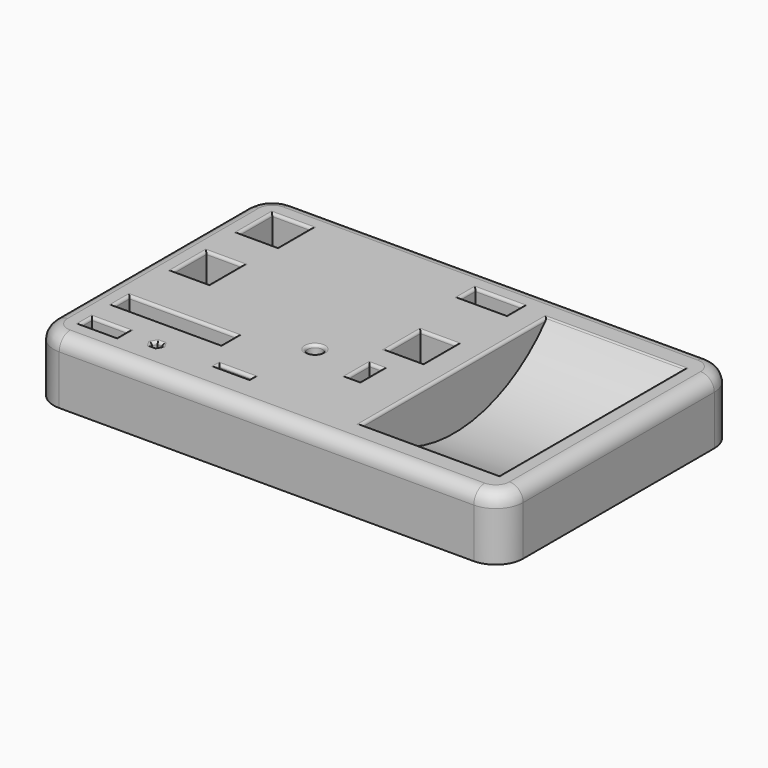
from build123d import *

# Parameters (mm, degrees)
F0_W          = 111
F0_H          = 107
F0_W_2        = 13
F0_H_2        = 5
F0_W_3        = 39
F0_H_3        = 7
F0_W_4        = 12
F0_H_4        = 1.5
F0_R          = 2.75
F0_W_5        = 4.5
F0_H_5        = 10
F0_H_6        = 15
F0_W_6        = 14
F0_W_7        = 17
F1_DEPTH      = 23
F2_W          = 111
F2_H          = 107
F3_DEPTH      = 3
F4_DEPTH      = 5
F5_DEPTH      = 13
F7_DEPTH      = 50
F9_DEPTH      = 10
F10_R         = 5
F11_T3_ANGLE  = 90
F11_T6_ANGLE  = 90
F11_T9_ANGLE  = 90
F11_T12_ANGLE = 90
F11_T15_DEPTH = 48
F11_T18_DEPTH = 48
F11_T21_DEPTH = 48
F11_T24_DEPTH = 48
F12_R         = 1


# Not quite as in the source:
# - a fillet or chamfer that OpenCascade refuses, or shapes differently, is made with other operations: its cross-section is extruded or revolved along the edge and cut away or added


with BuildPart() as f1:
    # F0 (on Top) → F1 (new body)
    with BuildSketch(Plane.XY):
        with Locations((55.5, 53.5)):
            Rectangle(F0_W, F0_H)
        with Locations((16.5, 12.5)):
            Rectangle(F0_W_2, F0_H_2, mode=Mode.SUBTRACT)
        Polygon((35.5980762114, 15), (36.4641016151, 13.5), (35.5980762114, 12), (33.8660254038, 12), (33, 13.5), (33.8660254038, 15), align=None, mode=Mode.SUBTRACT)
        with Locations((29.5, 28.5)):
            Rectangle(F0_W_3, F0_H_3, mode=Mode.SUBTRACT)
        with Locations((62.4641016151, 14.25)):
            Rectangle(F0_W_4, F0_H_4, mode=Mode.SUBTRACT)
        with Locations((71.75, 39.25)):
            Circle(F0_R, mode=Mode.SUBTRACT)
        with Locations((91.75, 37)):
            Rectangle(F0_W_5, F0_H_5, mode=Mode.SUBTRACT)
        with Locations((16.5, 59.5)):
            Rectangle(F0_W_2, F0_H_6, mode=Mode.SUBTRACT)
        with Locations((17, 89.5)):
            Rectangle(F0_W_6, F0_H_6, mode=Mode.SUBTRACT)
        with Locations((94.5, 59.5)):
            Rectangle(F0_W_2, F0_H_6, mode=Mode.SUBTRACT)
        with Locations((92.5, 93.5)):
            Rectangle(F0_W_7, F0_H_3, mode=Mode.SUBTRACT)
    extrude(amount=F1_DEPTH)

    # F2 (on face) → F3 (join)
    with BuildSketch(Plane(origin=(0, 0, 0), x_dir=(1, 0, 0), z_dir=(0, 0, -1))):
        with Locations((55.5, -53.5)):
            Rectangle(F2_W, F2_H)
    extrude(amount=-F3_DEPTH)

    # F4 (add): a face of the model
    f4_faces = [f1.faces().sort_by_distance(p)[0] for p in [
        (16.5, 12.5, 3),
    ]]
    extrude(f4_faces, amount=F4_DEPTH)

    # F5 (add): a face of the model
    f5_faces = [f1.faces().sort_by_distance(p)[0] for p in [
        (62.4641016151, 14.25, 3),
    ]]
    extrude(f5_faces, amount=F5_DEPTH)

    # F6 (on face) → F7 (join)
    with BuildSketch(Plane.YZ.offset(111)):
        with BuildLine():
            Line((11.0735931288, 23), (0, 23))
            Line((0, 23), (0, 0))
            Line((0, 0), (107, 0))
            Line((107, 0), (107, 23))
            Line((107, 23), (95.9264068712, 23))
            ThreePointArc((95.9264068712, 23), (53.5, 3), (11.0735931288, 23))
        make_face()
    extrude(amount=F7_DEPTH)

    # F8 (on face) → F9 (join)
    with BuildSketch(Plane.YZ.offset(161)):
        with BuildLine():
            Line((0, 23), (0, 0))
            Line((0, 0), (107, 0))
            Line((107, 0), (107, 23))
            Line((107, 23), (95.9264068712, 23))
            ThreePointArc((95.9264068712, 23), (53.5, 3), (11.0735931288, 23))
            Line((11.0735931288, 23), (0, 23))
        make_face()
        with BuildLine():
            Line((95.9264068712, 23), (11.0735931288, 23))
            ThreePointArc((11.0735931288, 23), (53.5, 3), (95.9264068712, 23))
        make_face()
    extrude(amount=F9_DEPTH)

    # F10
    f10_edges = [f1.edges().sort_by_distance(p)[0] for p in [
        (85.5, 107, 23),
        (171, 53.5, 23),
        (85.5, 0, 23),
        (0, 53.5, 23),
    ]]
    fillet(f10_edges, radius=F10_R)

    # F11: fillet of radius 10 on 4 edges, made by hand


with BuildPart() as f11_tool1:
    # F11_s2 → F11_t3 (revolve)
    with BuildSketch(Plane.YZ.offset(10)):
        with BuildLine():
            ThreePointArc((102, 23), (105.5355339059, 21.5355339059), (107, 18))
            Line((107, 18), (107, 23))
            Line((107, 23), (102, 23))
        make_face()
    revolve(axis=Axis((10, 97, 23), (0, 0, 1)), revolution_arc=F11_T3_ANGLE)


with BuildPart() as f11_tool4:
    # F11_s5 → F11_t6 (revolve)
    with BuildSketch(Plane.XZ.offset(-10)):
        with BuildLine():
            ThreePointArc((5, 23), (1.4644660941, 21.5355339059), (0, 18))
            Line((0, 18), (0, 23))
            Line((0, 23), (5, 23))
        make_face()
    revolve(axis=Axis((10, 10, 23), (0, 0, 1)), revolution_arc=F11_T6_ANGLE)


with BuildPart() as f11_tool7:
    # F11_s8 → F11_t9 (revolve)
    with BuildSketch(Plane.YZ.offset(161)):
        with BuildLine():
            ThreePointArc((5, 23), (1.4644660941, 21.5355339059), (0, 18))
            Line((0, 18), (0, 23))
            Line((0, 23), (5, 23))
        make_face()
    revolve(axis=Axis((161, 10, 23), (0, 0, 1)), revolution_arc=F11_T9_ANGLE)


with BuildPart() as f11_tool10:
    # F11_s11 → F11_t12 (revolve)
    with BuildSketch(Plane.XZ.offset(-97)):
        with BuildLine():
            ThreePointArc((166, 23), (169.5355339059, 21.5355339059), (171, 18))
            Line((171, 18), (171, 23))
            Line((171, 23), (166, 23))
        make_face()
    revolve(axis=Axis((161, 97, 23), (0, 0, 1)), revolution_arc=F11_T12_ANGLE)


with BuildPart() as f11_tool13:
    # F11_s14 → F11_t15 (new body)
    with BuildSketch(Plane.XY.offset(-25)):
        with BuildLine():
            ThreePointArc((161, 107), (168.0710678119, 104.0710678119), (171, 97))
            Line((171, 97), (171, 107))
            Line((171, 107), (161, 107))
        make_face()
    extrude(amount=F11_T15_DEPTH)


with BuildPart() as f11_tool16:
    # F11_s17 → F11_t18 (new body)
    with BuildSketch(Plane.XY.offset(23)):
        with BuildLine():
            ThreePointArc((161, 0), (168.0710678119, 2.9289321881), (171, 10))
            Line((171, 10), (171, 0))
            Line((171, 0), (161, 0))
        make_face()
    extrude(amount=-F11_T18_DEPTH)


with BuildPart() as f11_tool19:
    # F11_s20 → F11_t21 (new body)
    with BuildSketch(Plane.XY.offset(-25)):
        with BuildLine():
            ThreePointArc((0, 10), (2.9289321881, 2.9289321881), (10, 0))
            Line((10, 0), (0, 0))
            Line((0, 0), (0, 10))
        make_face()
    extrude(amount=F11_T21_DEPTH)


with BuildPart() as f11_tool22:
    # F11_s23 → F11_t24 (new body)
    with BuildSketch(Plane.XY.offset(23)):
        with BuildLine():
            ThreePointArc((0, 97), (2.9289321881, 104.0710678119), (10, 107))
            Line((10, 107), (0, 107))
            Line((0, 107), (0, 97))
        make_face()
    extrude(amount=-F11_T24_DEPTH)


with BuildPart() as f1_1:
    add(f1.part)

    # F11_t25: cut F11_tool1, F11_tool4, F11_tool7, F11_tool10, F11_tool13, F11_tool16, F11_tool19, F11_tool22
    add([f11_tool1.part, f11_tool4.part, f11_tool7.part, f11_tool10.part, f11_tool13.part, f11_tool16.part, f11_tool19.part, f11_tool22.part], mode=Mode.SUBTRACT)

    # F12
    f12_edges = [f1_1.edges().sort_by_distance(p)[0] for p in [
        (85.5, 102, 23),
        (164.535534, 100.535534, 23),
        (166, 53.5, 23),
        (164.535534, 6.464466, 23),
        (85.5, 5, 23),
        (6.464466, 6.464466, 23),
        (5, 53.5, 23),
        (6.464466, 100.535534, 23),
        (10, 12.5, 23),
        (16.5, 10, 23),
        (16.5, 15, 23),
        (23, 12.5, 23),
        (36.031089, 14.25, 23),
        (34.732051, 15, 23),
        (36.031089, 12.75, 23),
        (33.433013, 14.25, 23),
        (34.732051, 12, 23),
        (33.433013, 12.75, 23),
        (10, 28.5, 23),
        (29.5, 25, 23),
        (29.5, 32, 23),
        (49, 28.5, 23),
        (56.464102, 14.25, 23),
        (62.464102, 13.5, 23),
        (62.464102, 15, 23),
        (68.464102, 14.25, 23),
        (69, 39.25, 23),
        (89.5, 37, 23),
        (91.75, 32, 23),
        (91.75, 42, 23),
        (94, 37, 23),
        (136, 11.073593, 23),
        (111, 53.5, 23),
        (161, 53.5, 23),
        (136, 95.926407, 23),
        (10, 59.5, 23),
        (16.5, 52, 23),
        (16.5, 67, 23),
        (23, 59.5, 23),
        (17, 82, 23),
        (24, 89.5, 23),
        (10, 89.5, 23),
        (17, 97, 23),
        (94.5, 67, 23),
        (88, 59.5, 23),
        (101, 59.5, 23),
        (94.5, 52, 23),
        (92.5, 90, 23),
        (101, 93.5, 23),
        (84, 93.5, 23),
        (92.5, 97, 23),
    ]]
    fillet(f12_edges, radius=F12_R)


solid = f1_1.part
